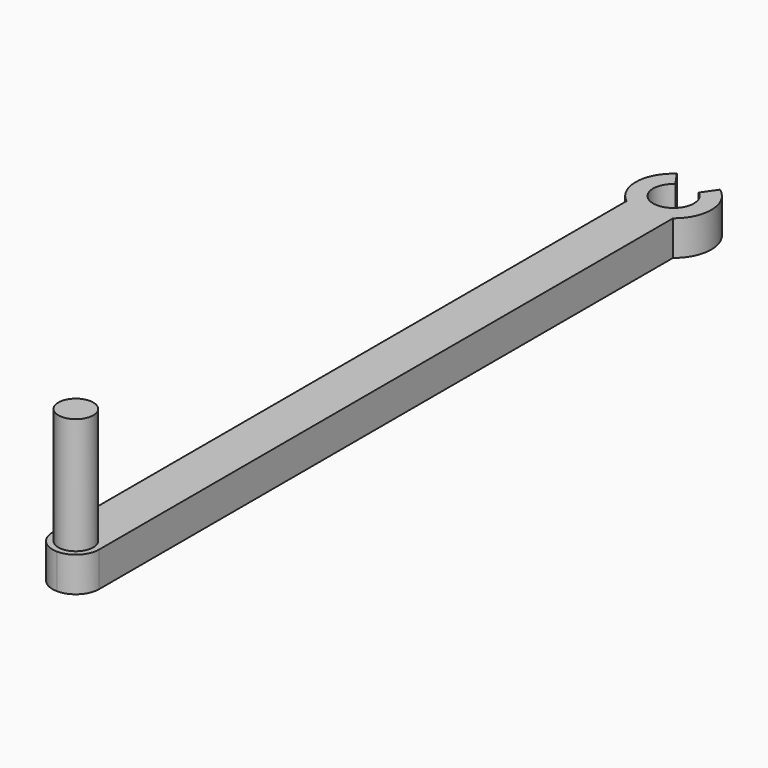
from build123d import *

# Parameters (mm, degrees)
F1_DEPTH = 3
F2_R     = 1.5
F3_DEPTH = 10


# Not quite as in the source:
# - a feature names something its author has since deleted; it is built from what else it names


with BuildPart() as f1:
    # F0 (on Top) → F1 (new body)
    with BuildSketch(Plane.XY):
        with BuildLine():
            ThreePointArc((3.25, 63.9241337907), (2.1924432633, 64.1010126169), (1.25, 64.6123960992))
            Line((1.25, 64.6123960992), (1.25, 2.9241337907))
            ThreePointArc((1.25, 2.9241337907), (1.8357864376, 4.338347353), (3.25, 4.9241337907))
            Line((3.25, 4.9241337907), (3.25, 63.9241337907))
        make_face()
        with BuildLine():
            ThreePointArc((3.25, 4.9241337907), (1.8357864376, 4.338347353), (1.25, 2.9241337907))
            ThreePointArc((1.25, 2.9241337907), (1.8357864376, 1.5099202283), (3.25, 0.9241337907))
            Line((3.25, 0.9241337907), (3.25, 4.9241337907))
        make_face()
        with BuildLine():
            ThreePointArc((5.25, 64.6123960992), (4.3075567367, 64.1010126169), (3.25, 63.9241337907))
            Line((3.25, 63.9241337907), (3.25, 4.9241337907))
            ThreePointArc((3.25, 4.9241337907), (4.6642135624, 4.338347353), (5.25, 2.9241337907))
            Line((5.25, 2.9241337907), (5.25, 64.6123960992))
        make_face()
        with BuildLine():
            ThreePointArc((5.25, 2.9241337907), (4.6642135624, 4.338347353), (3.25, 4.9241337907))
            Line((3.25, 4.9241337907), (3.25, 0.9241337907))
            ThreePointArc((3.25, 0.9241337907), (4.6642135624, 1.5099202283), (5.25, 2.9241337907))
        make_face()
        with BuildLine():
            Line((2.25, 68.6102744523), (1.3928571429, 69.8412521623))
            ThreePointArc((1.3928571429, 69.8412521623), (0.0012122742, 67.2628936507), (1.25, 64.6123960992))
            ThreePointArc((1.25, 64.6123960992), (2.1924432633, 64.1010126169), (3.25, 63.9241337907))
            ThreePointArc((3.25, 63.9241337907), (4.3075567367, 64.1010126169), (5.25, 64.6123960992))
            ThreePointArc((5.25, 64.6123960992), (6.4987877258, 67.2628936507), (5.1071428571, 69.8412521623))
            Line((5.1071428571, 69.8412521623), (4.25, 68.6102744523))
            ThreePointArc((4.25, 68.6102744523), (3.25, 65.4241337907), (2.25, 68.6102744523))
        make_face()
    extrude(amount=F1_DEPTH)

    # F2 (on face) → F3 (join)
    with BuildSketch(Plane.XY.offset(3)):
        with Locations((3.25, 2.9241337907)):
            Circle(F2_R)
    extrude(amount=F3_DEPTH)


solid = f1.part
